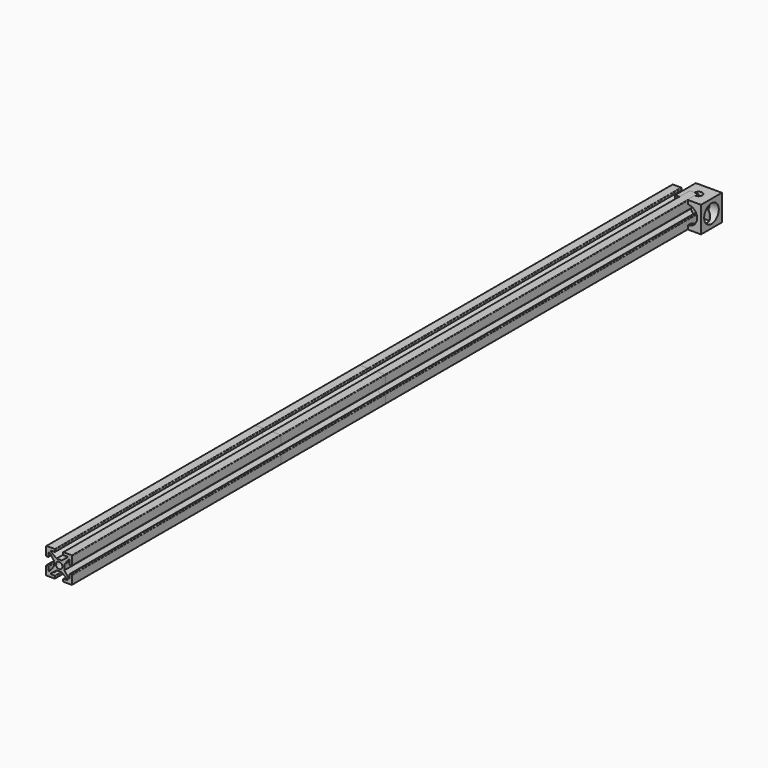
from build123d import *

# Parameters (mm, degrees)
F0_R      = 1.25
F1_DEPTH  = 300
F2_DEPTH  = 200
F3_W      = 10
F3_H      = 10
F4_DEPTH  = 10
F5_R      = 1.5
F6_DEPTH  = 305.001
F7_R      = 1.5
F8_DEPTH  = 10.001
F9_R      = 1.5
F10_DEPTH = 10.001
F11_R     = 3.5
F12_DEPTH = 7
F13_R     = 3.5
F14_DEPTH = 7
F15_R     = 3.5
F16_DEPTH = 7
F17_DEPTH = 100
F18_DEPTH = 150


with BuildPart() as f1:
    # F0 (on Front) → F1 (new body)
    with BuildSketch(Plane.XZ):
        with BuildLine():
            Line((1, 2), (-1, 2))
            Line((-1, 2), (-3.1201308818, 3.6418726247))
            ThreePointArc((-3.1201308818, 3.6418726247), (-3.1869163514, 3.8647090602), (-2.9976738151, 4))
            Line((-2.9976738151, 4), (-1.7, 4))
            ThreePointArc((-1.7, 4), (-1.5585786438, 4.0585786438), (-1.5, 4.2))
            Line((-1.5, 4.2), (-1.5, 4.8))
            ThreePointArc((-1.5, 4.8), (-1.5585786438, 4.9414213562), (-1.7, 5))
            Line((-1.7, 5), (-4.8, 5))
            ThreePointArc((-4.8, 5), (-4.9414213562, 4.9414213562), (-5, 4.8))
            Line((-5, 4.8), (-5, 1.7))
            ThreePointArc((-5, 1.7), (-4.9414213562, 1.5585786438), (-4.8, 1.5))
            Line((-4.8, 1.5), (-4.2, 1.5))
            ThreePointArc((-4.2, 1.5), (-4.0585786438, 1.5585786438), (-4, 1.7))
            Line((-4, 1.7), (-4, 2.9976738151))
            ThreePointArc((-4, 2.9976738151), (-3.8647090602, 3.1869163514), (-3.6418726247, 3.1201308818))
            Line((-3.6418726247, 3.1201308818), (-2, 1))
            Line((-2, 1), (-2, -1))
            Line((-2, -1), (-3.6418726247, -3.1201308818))
            ThreePointArc((-3.6418726247, -3.1201308818), (-3.8647090602, -3.1869163514), (-4, -2.9976738151))
            Line((-4, -2.9976738151), (-4, -1.7))
            ThreePointArc((-4, -1.7), (-4.0585786438, -1.5585786438), (-4.2, -1.5))
            Line((-4.2, -1.5), (-4.8, -1.5))
            ThreePointArc((-4.8, -1.5), (-4.9414213562, -1.5585786438), (-5, -1.7))
            Line((-5, -1.7), (-5, -4.8))
            ThreePointArc((-5, -4.8), (-4.9414213562, -4.9414213562), (-4.8, -5))
            Line((-4.8, -5), (-1.7, -5))
            ThreePointArc((-1.7, -5), (-1.5585786438, -4.9414213562), (-1.5, -4.8))
            Line((-1.5, -4.8), (-1.5, -4.2))
            ThreePointArc((-1.5, -4.2), (-1.5585786438, -4.0585786438), (-1.7, -4))
            Line((-1.7, -4), (-2.9976738151, -4))
            ThreePointArc((-2.9976738151, -4), (-3.1869163514, -3.8647090602), (-3.1201308818, -3.6418726247))
            Line((-3.1201308818, -3.6418726247), (-1, -2))
            Line((-1, -2), (1, -2))
            Line((1, -2), (3.1201308818, -3.6418726247))
            ThreePointArc((3.1201308818, -3.6418726247), (3.1869163514, -3.8647090602), (2.9976738151, -4))
            Line((2.9976738151, -4), (1.7, -4))
            ThreePointArc((1.7, -4), (1.5585786438, -4.0585786438), (1.5, -4.2))
            Line((1.5, -4.2), (1.5, -4.8))
            ThreePointArc((1.5, -4.8), (1.5585786438, -4.9414213562), (1.7, -5))
            Line((1.7, -5), (4.8, -5))
            ThreePointArc((4.8, -5), (4.9414213562, -4.9414213562), (5, -4.8))
            Line((5, -4.8), (5, -1.7))
            ThreePointArc((5, -1.7), (4.9414213562, -1.5585786438), (4.8, -1.5))
            Line((4.8, -1.5), (4.2, -1.5))
            ThreePointArc((4.2, -1.5), (4.0585786438, -1.5585786438), (4, -1.7))
            Line((4, -1.7), (4, -2.9976738151))
            ThreePointArc((4, -2.9976738151), (3.8647090602, -3.1869163514), (3.6418726247, -3.1201308818))
            Line((3.6418726247, -3.1201308818), (2, -1))
            Line((2, -1), (2, 1))
            Line((2, 1), (3.6418726247, 3.1201308818))
            ThreePointArc((3.6418726247, 3.1201308818), (3.8647090602, 3.1869163514), (4, 2.9976738151))
            Line((4, 2.9976738151), (4, 1.7))
            ThreePointArc((4, 1.7), (4.0585786438, 1.5585786438), (4.2, 1.5))
            Line((4.2, 1.5), (4.8, 1.5))
            ThreePointArc((4.8, 1.5), (4.9414213562, 1.5585786438), (5, 1.7))
            Line((5, 1.7), (5, 4.8))
            ThreePointArc((5, 4.8), (4.9414213562, 4.9414213562), (4.8, 5))
            Line((4.8, 5), (1.7, 5))
            ThreePointArc((1.7, 5), (1.5585786438, 4.9414213562), (1.5, 4.8))
            Line((1.5, 4.8), (1.5, 4.2))
            ThreePointArc((1.5, 4.2), (1.5585786438, 4.0585786438), (1.7, 4))
            Line((1.7, 4), (2.9976738151, 4))
            ThreePointArc((2.9976738151, 4), (3.1869163514, 3.8647090602), (3.1201308818, 3.6418726247))
            Line((3.1201308818, 3.6418726247), (1, 2))
        make_face()
        Circle(F0_R, mode=Mode.SUBTRACT)
    extrude(amount=F1_DEPTH)


with BuildPart() as f2:
    # F0 (on Front) → F2 (new body)
    with BuildSketch(Plane.XZ):
        with BuildLine():
            Line((1, 2), (-1, 2))
            Line((-1, 2), (-3.1201308818, 3.6418726247))
            ThreePointArc((-3.1201308818, 3.6418726247), (-3.1869163514, 3.8647090602), (-2.9976738151, 4))
            Line((-2.9976738151, 4), (-1.7, 4))
            ThreePointArc((-1.7, 4), (-1.5585786438, 4.0585786438), (-1.5, 4.2))
            Line((-1.5, 4.2), (-1.5, 4.8))
            ThreePointArc((-1.5, 4.8), (-1.5585786438, 4.9414213562), (-1.7, 5))
            Line((-1.7, 5), (-4.8, 5))
            ThreePointArc((-4.8, 5), (-4.9414213562, 4.9414213562), (-5, 4.8))
            Line((-5, 4.8), (-5, 1.7))
            ThreePointArc((-5, 1.7), (-4.9414213562, 1.5585786438), (-4.8, 1.5))
            Line((-4.8, 1.5), (-4.2, 1.5))
            ThreePointArc((-4.2, 1.5), (-4.0585786438, 1.5585786438), (-4, 1.7))
            Line((-4, 1.7), (-4, 2.9976738151))
            ThreePointArc((-4, 2.9976738151), (-3.8647090602, 3.1869163514), (-3.6418726247, 3.1201308818))
            Line((-3.6418726247, 3.1201308818), (-2, 1))
            Line((-2, 1), (-2, -1))
            Line((-2, -1), (-3.6418726247, -3.1201308818))
            ThreePointArc((-3.6418726247, -3.1201308818), (-3.8647090602, -3.1869163514), (-4, -2.9976738151))
            Line((-4, -2.9976738151), (-4, -1.7))
            ThreePointArc((-4, -1.7), (-4.0585786438, -1.5585786438), (-4.2, -1.5))
            Line((-4.2, -1.5), (-4.8, -1.5))
            ThreePointArc((-4.8, -1.5), (-4.9414213562, -1.5585786438), (-5, -1.7))
            Line((-5, -1.7), (-5, -4.8))
            ThreePointArc((-5, -4.8), (-4.9414213562, -4.9414213562), (-4.8, -5))
            Line((-4.8, -5), (-1.7, -5))
            ThreePointArc((-1.7, -5), (-1.5585786438, -4.9414213562), (-1.5, -4.8))
            Line((-1.5, -4.8), (-1.5, -4.2))
            ThreePointArc((-1.5, -4.2), (-1.5585786438, -4.0585786438), (-1.7, -4))
            Line((-1.7, -4), (-2.9976738151, -4))
            ThreePointArc((-2.9976738151, -4), (-3.1869163514, -3.8647090602), (-3.1201308818, -3.6418726247))
            Line((-3.1201308818, -3.6418726247), (-1, -2))
            Line((-1, -2), (1, -2))
            Line((1, -2), (3.1201308818, -3.6418726247))
            ThreePointArc((3.1201308818, -3.6418726247), (3.1869163514, -3.8647090602), (2.9976738151, -4))
            Line((2.9976738151, -4), (1.7, -4))
            ThreePointArc((1.7, -4), (1.5585786438, -4.0585786438), (1.5, -4.2))
            Line((1.5, -4.2), (1.5, -4.8))
            ThreePointArc((1.5, -4.8), (1.5585786438, -4.9414213562), (1.7, -5))
            Line((1.7, -5), (4.8, -5))
            ThreePointArc((4.8, -5), (4.9414213562, -4.9414213562), (5, -4.8))
            Line((5, -4.8), (5, -1.7))
            ThreePointArc((5, -1.7), (4.9414213562, -1.5585786438), (4.8, -1.5))
            Line((4.8, -1.5), (4.2, -1.5))
            ThreePointArc((4.2, -1.5), (4.0585786438, -1.5585786438), (4, -1.7))
            Line((4, -1.7), (4, -2.9976738151))
            ThreePointArc((4, -2.9976738151), (3.8647090602, -3.1869163514), (3.6418726247, -3.1201308818))
            Line((3.6418726247, -3.1201308818), (2, -1))
            Line((2, -1), (2, 1))
            Line((2, 1), (3.6418726247, 3.1201308818))
            ThreePointArc((3.6418726247, 3.1201308818), (3.8647090602, 3.1869163514), (4, 2.9976738151))
            Line((4, 2.9976738151), (4, 1.7))
            ThreePointArc((4, 1.7), (4.0585786438, 1.5585786438), (4.2, 1.5))
            Line((4.2, 1.5), (4.8, 1.5))
            ThreePointArc((4.8, 1.5), (4.9414213562, 1.5585786438), (5, 1.7))
            Line((5, 1.7), (5, 4.8))
            ThreePointArc((5, 4.8), (4.9414213562, 4.9414213562), (4.8, 5))
            Line((4.8, 5), (1.7, 5))
            ThreePointArc((1.7, 5), (1.5585786438, 4.9414213562), (1.5, 4.8))
            Line((1.5, 4.8), (1.5, 4.2))
            ThreePointArc((1.5, 4.2), (1.5585786438, 4.0585786438), (1.7, 4))
            Line((1.7, 4), (2.9976738151, 4))
            ThreePointArc((2.9976738151, 4), (3.1869163514, 3.8647090602), (3.1201308818, 3.6418726247))
            Line((3.1201308818, 3.6418726247), (1, 2))
        make_face()
        Circle(F0_R, mode=Mode.SUBTRACT)
    extrude(amount=F2_DEPTH)


with BuildPart() as f4:
    # F3 (on Right) → F4 (new body)
    with BuildSketch(Plane.YZ):
        Rectangle(F3_W, F3_H)
    extrude(amount=F4_DEPTH)

    # F5 (on face) → F6 (cut, through all)
    with BuildSketch(Plane(origin=(0, 5, 0), x_dir=(-1, 0, 0), z_dir=(0, 1, 0))):
        with Locations((-5, 0)):
            Circle(F5_R)
    extrude(amount=-F6_DEPTH, mode=Mode.SUBTRACT)

    # F7 (on face) → F8 (cut, through all)
    with BuildSketch(Plane.XY.offset(5)):
        with Locations((5, 0)):
            Circle(F7_R)
    extrude(amount=-F8_DEPTH, mode=Mode.SUBTRACT)

    # F9 (on face) → F10 (cut, through all)
    with BuildSketch(Plane(origin=(0, 0, 0), x_dir=(0, -1, 0), z_dir=(-1, 0, 0))):
        Circle(F9_R)
    extrude(amount=-F10_DEPTH, mode=Mode.SUBTRACT)

    # F11 (on face) → F12 (cut)
    with BuildSketch(Plane.XZ.offset(5)):
        with Locations((5, 0)):
            Circle(F11_R)
    extrude(amount=-F12_DEPTH, mode=Mode.SUBTRACT)

    # F13 (on face) → F14 (cut)
    with BuildSketch(Plane(origin=(0, 0, -5), x_dir=(1, 0, 0), z_dir=(0, 0, -1))):
        with Locations((5, 0)):
            Circle(F13_R)
    extrude(amount=-F14_DEPTH, mode=Mode.SUBTRACT)

    # F15 (on face) → F16 (cut)
    with BuildSketch(Plane.YZ.offset(10)):
        Circle(F15_R)
    extrude(amount=-F16_DEPTH, mode=Mode.SUBTRACT)


with BuildPart() as f17:
    # F0 (on Front) → F17 (new body)
    with BuildSketch(Plane.XZ):
        with BuildLine():
            Line((1, 2), (-1, 2))
            Line((-1, 2), (-3.1201308818, 3.6418726247))
            ThreePointArc((-3.1201308818, 3.6418726247), (-3.1869163514, 3.8647090602), (-2.9976738151, 4))
            Line((-2.9976738151, 4), (-1.7, 4))
            ThreePointArc((-1.7, 4), (-1.5585786438, 4.0585786438), (-1.5, 4.2))
            Line((-1.5, 4.2), (-1.5, 4.8))
            ThreePointArc((-1.5, 4.8), (-1.5585786438, 4.9414213562), (-1.7, 5))
            Line((-1.7, 5), (-4.8, 5))
            ThreePointArc((-4.8, 5), (-4.9414213562, 4.9414213562), (-5, 4.8))
            Line((-5, 4.8), (-5, 1.7))
            ThreePointArc((-5, 1.7), (-4.9414213562, 1.5585786438), (-4.8, 1.5))
            Line((-4.8, 1.5), (-4.2, 1.5))
            ThreePointArc((-4.2, 1.5), (-4.0585786438, 1.5585786438), (-4, 1.7))
            Line((-4, 1.7), (-4, 2.9976738151))
            ThreePointArc((-4, 2.9976738151), (-3.8647090602, 3.1869163514), (-3.6418726247, 3.1201308818))
            Line((-3.6418726247, 3.1201308818), (-2, 1))
            Line((-2, 1), (-2, -1))
            Line((-2, -1), (-3.6418726247, -3.1201308818))
            ThreePointArc((-3.6418726247, -3.1201308818), (-3.8647090602, -3.1869163514), (-4, -2.9976738151))
            Line((-4, -2.9976738151), (-4, -1.7))
            ThreePointArc((-4, -1.7), (-4.0585786438, -1.5585786438), (-4.2, -1.5))
            Line((-4.2, -1.5), (-4.8, -1.5))
            ThreePointArc((-4.8, -1.5), (-4.9414213562, -1.5585786438), (-5, -1.7))
            Line((-5, -1.7), (-5, -4.8))
            ThreePointArc((-5, -4.8), (-4.9414213562, -4.9414213562), (-4.8, -5))
            Line((-4.8, -5), (-1.7, -5))
            ThreePointArc((-1.7, -5), (-1.5585786438, -4.9414213562), (-1.5, -4.8))
            Line((-1.5, -4.8), (-1.5, -4.2))
            ThreePointArc((-1.5, -4.2), (-1.5585786438, -4.0585786438), (-1.7, -4))
            Line((-1.7, -4), (-2.9976738151, -4))
            ThreePointArc((-2.9976738151, -4), (-3.1869163514, -3.8647090602), (-3.1201308818, -3.6418726247))
            Line((-3.1201308818, -3.6418726247), (-1, -2))
            Line((-1, -2), (1, -2))
            Line((1, -2), (3.1201308818, -3.6418726247))
            ThreePointArc((3.1201308818, -3.6418726247), (3.1869163514, -3.8647090602), (2.9976738151, -4))
            Line((2.9976738151, -4), (1.7, -4))
            ThreePointArc((1.7, -4), (1.5585786438, -4.0585786438), (1.5, -4.2))
            Line((1.5, -4.2), (1.5, -4.8))
            ThreePointArc((1.5, -4.8), (1.5585786438, -4.9414213562), (1.7, -5))
            Line((1.7, -5), (4.8, -5))
            ThreePointArc((4.8, -5), (4.9414213562, -4.9414213562), (5, -4.8))
            Line((5, -4.8), (5, -1.7))
            ThreePointArc((5, -1.7), (4.9414213562, -1.5585786438), (4.8, -1.5))
            Line((4.8, -1.5), (4.2, -1.5))
            ThreePointArc((4.2, -1.5), (4.0585786438, -1.5585786438), (4, -1.7))
            Line((4, -1.7), (4, -2.9976738151))
            ThreePointArc((4, -2.9976738151), (3.8647090602, -3.1869163514), (3.6418726247, -3.1201308818))
            Line((3.6418726247, -3.1201308818), (2, -1))
            Line((2, -1), (2, 1))
            Line((2, 1), (3.6418726247, 3.1201308818))
            ThreePointArc((3.6418726247, 3.1201308818), (3.8647090602, 3.1869163514), (4, 2.9976738151))
            Line((4, 2.9976738151), (4, 1.7))
            ThreePointArc((4, 1.7), (4.0585786438, 1.5585786438), (4.2, 1.5))
            Line((4.2, 1.5), (4.8, 1.5))
            ThreePointArc((4.8, 1.5), (4.9414213562, 1.5585786438), (5, 1.7))
            Line((5, 1.7), (5, 4.8))
            ThreePointArc((5, 4.8), (4.9414213562, 4.9414213562), (4.8, 5))
            Line((4.8, 5), (1.7, 5))
            ThreePointArc((1.7, 5), (1.5585786438, 4.9414213562), (1.5, 4.8))
            Line((1.5, 4.8), (1.5, 4.2))
            ThreePointArc((1.5, 4.2), (1.5585786438, 4.0585786438), (1.7, 4))
            Line((1.7, 4), (2.9976738151, 4))
            ThreePointArc((2.9976738151, 4), (3.1869163514, 3.8647090602), (3.1201308818, 3.6418726247))
            Line((3.1201308818, 3.6418726247), (1, 2))
        make_face()
        Circle(F0_R, mode=Mode.SUBTRACT)
    extrude(amount=F17_DEPTH)


with BuildPart() as f18:
    # F0 (on Front) → F18 (new body)
    with BuildSketch(Plane.XZ):
        with BuildLine():
            Line((1, 2), (-1, 2))
            Line((-1, 2), (-3.1201308818, 3.6418726247))
            ThreePointArc((-3.1201308818, 3.6418726247), (-3.1869163514, 3.8647090602), (-2.9976738151, 4))
            Line((-2.9976738151, 4), (-1.7, 4))
            ThreePointArc((-1.7, 4), (-1.5585786438, 4.0585786438), (-1.5, 4.2))
            Line((-1.5, 4.2), (-1.5, 4.8))
            ThreePointArc((-1.5, 4.8), (-1.5585786438, 4.9414213562), (-1.7, 5))
            Line((-1.7, 5), (-4.8, 5))
            ThreePointArc((-4.8, 5), (-4.9414213562, 4.9414213562), (-5, 4.8))
            Line((-5, 4.8), (-5, 1.7))
            ThreePointArc((-5, 1.7), (-4.9414213562, 1.5585786438), (-4.8, 1.5))
            Line((-4.8, 1.5), (-4.2, 1.5))
            ThreePointArc((-4.2, 1.5), (-4.0585786438, 1.5585786438), (-4, 1.7))
            Line((-4, 1.7), (-4, 2.9976738151))
            ThreePointArc((-4, 2.9976738151), (-3.8647090602, 3.1869163514), (-3.6418726247, 3.1201308818))
            Line((-3.6418726247, 3.1201308818), (-2, 1))
            Line((-2, 1), (-2, -1))
            Line((-2, -1), (-3.6418726247, -3.1201308818))
            ThreePointArc((-3.6418726247, -3.1201308818), (-3.8647090602, -3.1869163514), (-4, -2.9976738151))
            Line((-4, -2.9976738151), (-4, -1.7))
            ThreePointArc((-4, -1.7), (-4.0585786438, -1.5585786438), (-4.2, -1.5))
            Line((-4.2, -1.5), (-4.8, -1.5))
            ThreePointArc((-4.8, -1.5), (-4.9414213562, -1.5585786438), (-5, -1.7))
            Line((-5, -1.7), (-5, -4.8))
            ThreePointArc((-5, -4.8), (-4.9414213562, -4.9414213562), (-4.8, -5))
            Line((-4.8, -5), (-1.7, -5))
            ThreePointArc((-1.7, -5), (-1.5585786438, -4.9414213562), (-1.5, -4.8))
            Line((-1.5, -4.8), (-1.5, -4.2))
            ThreePointArc((-1.5, -4.2), (-1.5585786438, -4.0585786438), (-1.7, -4))
            Line((-1.7, -4), (-2.9976738151, -4))
            ThreePointArc((-2.9976738151, -4), (-3.1869163514, -3.8647090602), (-3.1201308818, -3.6418726247))
            Line((-3.1201308818, -3.6418726247), (-1, -2))
            Line((-1, -2), (1, -2))
            Line((1, -2), (3.1201308818, -3.6418726247))
            ThreePointArc((3.1201308818, -3.6418726247), (3.1869163514, -3.8647090602), (2.9976738151, -4))
            Line((2.9976738151, -4), (1.7, -4))
            ThreePointArc((1.7, -4), (1.5585786438, -4.0585786438), (1.5, -4.2))
            Line((1.5, -4.2), (1.5, -4.8))
            ThreePointArc((1.5, -4.8), (1.5585786438, -4.9414213562), (1.7, -5))
            Line((1.7, -5), (4.8, -5))
            ThreePointArc((4.8, -5), (4.9414213562, -4.9414213562), (5, -4.8))
            Line((5, -4.8), (5, -1.7))
            ThreePointArc((5, -1.7), (4.9414213562, -1.5585786438), (4.8, -1.5))
            Line((4.8, -1.5), (4.2, -1.5))
            ThreePointArc((4.2, -1.5), (4.0585786438, -1.5585786438), (4, -1.7))
            Line((4, -1.7), (4, -2.9976738151))
            ThreePointArc((4, -2.9976738151), (3.8647090602, -3.1869163514), (3.6418726247, -3.1201308818))
            Line((3.6418726247, -3.1201308818), (2, -1))
            Line((2, -1), (2, 1))
            Line((2, 1), (3.6418726247, 3.1201308818))
            ThreePointArc((3.6418726247, 3.1201308818), (3.8647090602, 3.1869163514), (4, 2.9976738151))
            Line((4, 2.9976738151), (4, 1.7))
            ThreePointArc((4, 1.7), (4.0585786438, 1.5585786438), (4.2, 1.5))
            Line((4.2, 1.5), (4.8, 1.5))
            ThreePointArc((4.8, 1.5), (4.9414213562, 1.5585786438), (5, 1.7))
            Line((5, 1.7), (5, 4.8))
            ThreePointArc((5, 4.8), (4.9414213562, 4.9414213562), (4.8, 5))
            Line((4.8, 5), (1.7, 5))
            ThreePointArc((1.7, 5), (1.5585786438, 4.9414213562), (1.5, 4.8))
            Line((1.5, 4.8), (1.5, 4.2))
            ThreePointArc((1.5, 4.2), (1.5585786438, 4.0585786438), (1.7, 4))
            Line((1.7, 4), (2.9976738151, 4))
            ThreePointArc((2.9976738151, 4), (3.1869163514, 3.8647090602), (3.1201308818, 3.6418726247))
            Line((3.1201308818, 3.6418726247), (1, 2))
        make_face()
        Circle(F0_R, mode=Mode.SUBTRACT)
    extrude(amount=F18_DEPTH)


solid = Compound([f1.part, f2.part, f4.part, f17.part, f18.part])
